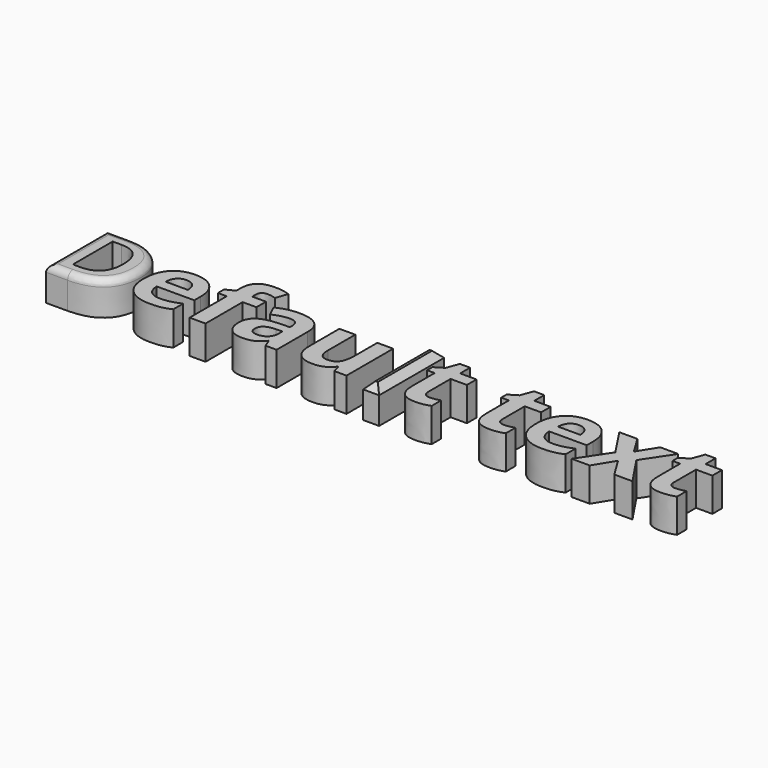
from build123d import *

# Parameters (mm, degrees)
F0_TEXT_SIZE = 80.4844053669
F1_DEPTH     = 25.4
F2_R         = 5.08
F3_SIZE      = 5.08


# Not quite as in the source:
# - Text() gives the source's letters only with a copy of the font that has no kerning and outlines rounded to 1/6400 em; it was checked with that copy


with BuildPart() as f1:
    # F0 (on Top) → F1 (new body)
    with BuildSketch(Plane.XY):
        with Locations((-115.8047094941, -28.3465869725)):
            Text('Default text', F0_TEXT_SIZE, font='Open Sans', font_style=FontStyle.BOLD, text_align=(TextAlign.LEFT, TextAlign.BOTTOM))
    extrude(amount=F1_DEPTH)

    # F2
    f2_edges = [f1.edges().sort_by_distance(p)[0] for p in [
        (-108.573689, 0.382573, 25.4),
        (-100.437218, -28.346587, 25.4),
    ]]
    fillet(f2_edges, radius=F2_R)

    # F3
    f3_edges = [f1.edges().sort_by_distance(p)[0] for p in [
        (142.273567, 2.231199, 25.4),
        (136.281251, 32.808985, 25.4),
        (130.288936, 2.231199, 25.4),
        (136.281251, -28.346587, 25.4),
    ]]
    chamfer(f3_edges, length=F3_SIZE)


solid = f1.part
